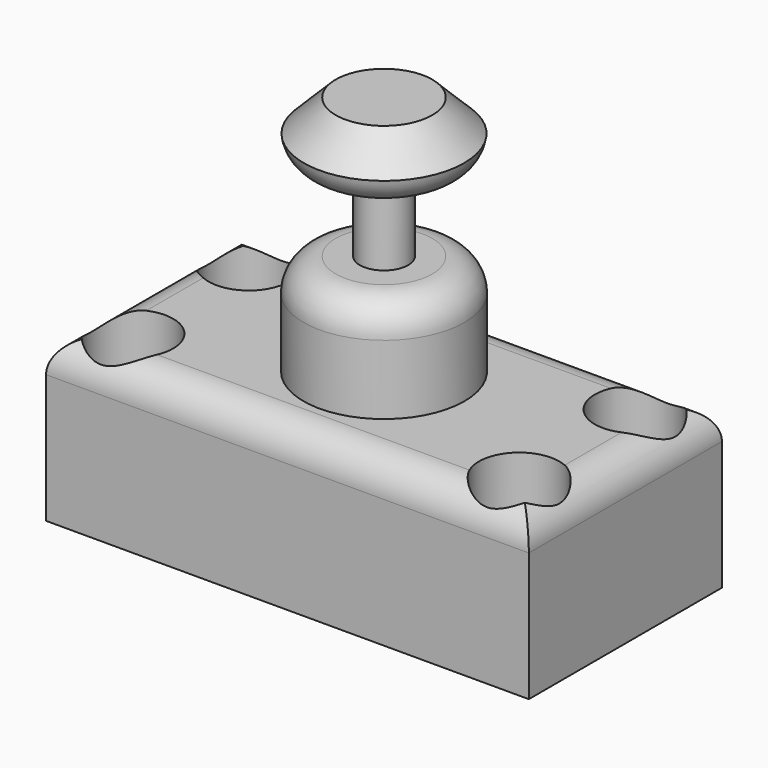
from build123d import *

# Parameters (mm, degrees)
F0_W        = 76.2
F0_H        = 38.1
F1_DEPTH    = 25.4
F2_R        = 6.35
F3_DEPTH    = 25.4
F4_R        = 12.7
F5_DEPTH    = 38.1
F6_W        = 12.7
F6_H        = 12.7
F8_T1_DEPTH = 101.6
F8_T3_DEPTH = 63.5


# Not quite as in the source:
# - a fillet or chamfer that OpenCascade refuses, or shapes differently, is made with other operations: its cross-section is extruded or revolved along the edge and cut away or added


with BuildPart() as f1:
    # F0 (on Top) → F1 (new body)
    with BuildSketch(Plane.XY):
        Rectangle(F0_W, F0_H)
    extrude(amount=F1_DEPTH)

    # F2 (on face) → F3 (cut)
    with BuildSketch(Plane.XY.offset(25.4)):
        with Locations((-30.48, 11.43)):
            Circle(F2_R)
        with Locations((-30.48, -11.43)):
            Circle(F2_R)
        with Locations((30.48, 11.43)):
            Circle(F2_R)
        with Locations((30.48, -11.43)):
            Circle(F2_R)
    extrude(amount=-F3_DEPTH, mode=Mode.SUBTRACT)

    # F4 (on face) → F5 (join)
    with BuildSketch(Plane.XY.offset(25.4)):
        Circle(F4_R)
    extrude(amount=F5_DEPTH)

    # F6 (on Front) → F7 (revolve, cut)
    with BuildSketch(Plane.XZ):
        with Locations((-10.1681923658, 47.7745333523)):
            Rectangle(F6_W, F6_H)
    revolve(axis=Axis((0, 0, 63.5), (0, 0, 1)), mode=Mode.SUBTRACT)

    # F8: fillet of radius 5.08 on 6 edges, made by hand

    # F8_s2 → F8_t1 (cut)
    with BuildSketch(Plane.YZ.offset(-50.8)):
        with BuildLine():
            ThreePointArc((-13.97, 25.4), (-17.5621024484, 23.9121024484), (-19.05, 20.32))
            Line((-19.05, 20.32), (-19.05, 25.4))
            Line((-19.05, 25.4), (-13.97, 25.4))
        make_face()
        with BuildLine():
            ThreePointArc((19.05, 20.32), (17.5621024484, 23.9121024484), (13.97, 25.4))
            Line((13.97, 25.4), (19.05, 25.4))
            Line((19.05, 25.4), (19.05, 20.32))
        make_face()
    extrude(amount=F8_T1_DEPTH, mode=Mode.SUBTRACT)

    # F8_s4 → F8_t3 (cut)
    with BuildSketch(Plane.XZ.offset(-31.75)):
        with BuildLine():
            ThreePointArc((-38.1, 20.32), (-36.6121024484, 23.9121024484), (-33.02, 25.4))
            Line((-33.02, 25.4), (-38.1, 25.4))
            Line((-38.1, 25.4), (-38.1, 20.32))
        make_face()
        with BuildLine():
            ThreePointArc((38.1, 20.32), (36.6121024484, 23.9121024484), (33.02, 25.4))
            Line((33.02, 25.4), (38.1, 25.4))
            Line((38.1, 25.4), (38.1, 20.32))
        make_face()
    extrude(amount=F8_T3_DEPTH, mode=Mode.SUBTRACT)

    # F8_s5 → F8_t6 (revolve, cut)
    with BuildSketch(Plane.XZ):
        with BuildLine():
            ThreePointArc((12.7, 36.3445333523), (11.2121024484, 39.9366358007), (7.62, 41.4245333523))
            Line((7.62, 41.4245333523), (12.7, 41.4245333523))
            Line((12.7, 41.4245333523), (12.7, 36.3445333523))
        make_face()
    revolve(axis=Axis((0, 0, 41.4245333523), (0, 0, -1)), mode=Mode.SUBTRACT)

    # F8_s7 → F8_t8 (revolve, cut)
    with BuildSketch(Plane.XZ):
        with BuildLine():
            ThreePointArc((7.62, 54.1245333523), (11.2121024484, 55.6124309038), (12.7, 59.2045333523))
            Line((12.7, 59.2045333523), (12.7, 54.1245333523))
            Line((12.7, 54.1245333523), (7.62, 54.1245333523))
        make_face()
    revolve(axis=Axis((0, 0, 54.1245333523), (0, 0, -1)), mode=Mode.SUBTRACT)

    # F9: chamfer of 5.08 on 1 edges, made by hand

    # F9_s1 → F9_t2 (revolve, cut)
    with BuildSketch(Plane.XZ):
        Polygon((12.7, 58.42), (7.62, 63.5), (12.7, 63.5), align=None)
    revolve(axis=Axis((0, 0, 63.5), (0, 0, 1)), mode=Mode.SUBTRACT)


solid = f1.part
